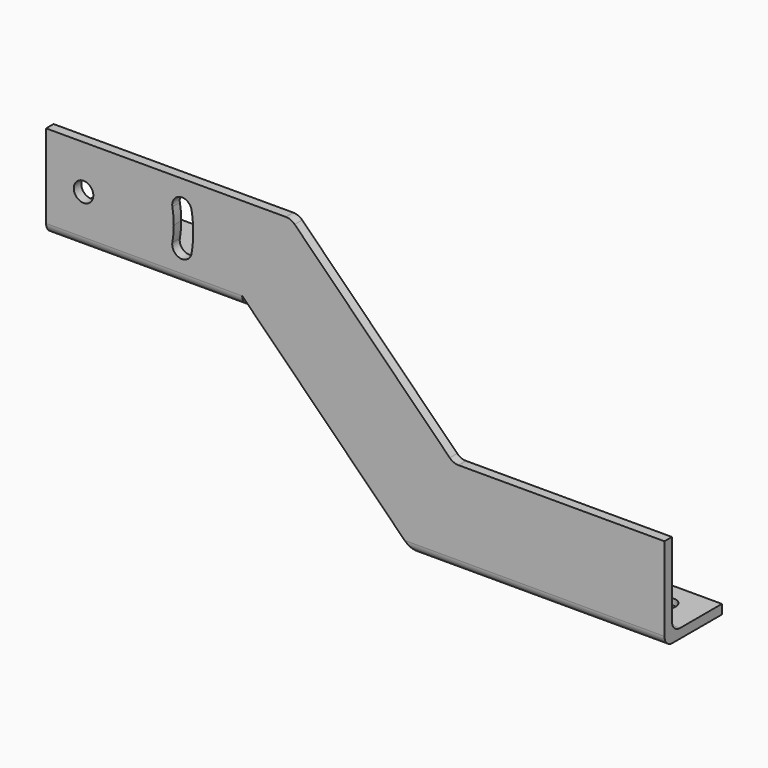
from build123d import *

# Parameters (mm, degrees)
F0_R        = 4.96062
F1_DEPTH    = 4.7625
F2_W        = 31.75
F2_H        = 4.7625
F3_DEPTH    = 127
F4_T1_DEPTH = 127
F4_T3_DEPTH = 152.4
F5_R        = 4.96062
F6_DEPTH    = 3.175
F7_W        = 31.75
F7_H        = 4.7625
F8_DEPTH    = 99.695
F9_R        = 5.08
F11_DEPTH   = 25.4


# Not quite as in the source:
# - a fillet or chamfer that OpenCascade refuses, or shapes differently, is made with other operations: its cross-section is extruded or revolved along the edge and cut away or added


with BuildPart() as f1:
    # F0 (on Front) → F1 (new body)
    with BuildSketch(Plane.XZ):
        with BuildLine():
            Line((-82.55, 82.55), (0, 0))
            Line((0, 0), (127, 0))
            Line((127, 0), (127, 47.625))
            Line((127, 47.625), (22.3571770291, 47.625))
            ThreePointArc((22.3571770291, 47.625), (19.9271372336, 48.1083649686), (17.8670489686, 49.4848719395))
            Line((17.8670489686, 49.4848719395), (-60.9632071525, 128.3151280605))
            ThreePointArc((-60.9632071525, 128.3151280605), (-63.0232954175, 129.6916350314), (-65.4533352131, 130.175))
            Line((-65.4533352131, 130.175), (-187.325, 130.175))
            Line((-187.325, 130.175), (-187.325, 82.55))
            Line((-187.325, 82.55), (-82.55, 82.55))
        make_face()
        with Locations((-168.275, 107.95)):
            Circle(F0_R, mode=Mode.SUBTRACT)
        with BuildLine():
            ThreePointArc((-113.3757178125, 117.6693530802), (-112.7358395418, 112.8283875), (-112.522, 107.95))
            ThreePointArc((-112.522, 107.95), (-112.7358395418, 103.0716125), (-113.3757178125, 98.2306469198))
            ThreePointArc((-113.3757178125, 98.2306469198), (-119.1163255014, 94.2169402337), (-123.1300321875, 99.9575479227))
            ThreePointArc((-123.1300321875, 99.9575479227), (-122.6038452724, 103.9383875), (-122.428, 107.95))
            ThreePointArc((-122.428, 107.95), (-122.6038452724, 111.9616125), (-123.1300321875, 115.9424520773))
            ThreePointArc((-123.1300321875, 115.9424520773), (-119.1163255014, 121.6830597663), (-113.3757178125, 117.6693530802))
        make_face(mode=Mode.SUBTRACT)
    extrude(amount=F1_DEPTH)

    # F2 (on face) → F3 (join)
    with BuildSketch(Plane.YZ.offset(127)):
        with Locations((15.875, 2.38125)):
            Rectangle(F2_W, F2_H)
    extrude(amount=-F3_DEPTH)

    # F4: fillet of radius 5.08 on 2 edges, made by hand

    # F4_s2 → F4_t1 (join)
    with BuildSketch(Plane.YZ):
        with BuildLine():
            ThreePointArc((5.08, 4.7625), (1.4878975516, 6.2503975516), (0, 9.8425))
            Line((0, 9.8425), (0, 4.7625))
            Line((0, 4.7625), (5.08, 4.7625))
        make_face()
    extrude(amount=F4_T1_DEPTH)

    # F4_s4 → F4_t3 (cut)
    with BuildSketch(Plane.YZ.offset(-12.7)):
        with BuildLine():
            ThreePointArc((-4.7625, 5.08), (-3.2746024484, 1.4878975516), (0.3175, 0))
            Line((0.3175, 0), (-4.7625, 0))
            Line((-4.7625, 0), (-4.7625, 5.08))
        make_face()
    extrude(amount=F4_T3_DEPTH, mode=Mode.SUBTRACT)

    # F5 (on face) → F6 (cut)
    with BuildSketch(Plane.XY.offset(4.7625)):
        with Locations((17.79778, 18.42008)):
            Circle(F5_R)
        with Locations((63.51778, 18.42008)):
            Circle(F5_R)
        with Locations((109.23778, 18.42008)):
            Circle(F5_R)
    extrude(amount=-F6_DEPTH, mode=Mode.SUBTRACT)

    # F7 (on face) → F8 (join)
    with BuildSketch(Plane(origin=(-187.325, 0, 0), x_dir=(0, -1, 0), z_dir=(-1, 0, 0))):
        with Locations((-15.875, 84.93125)):
            Rectangle(F7_W, F7_H)
    extrude(amount=-F8_DEPTH)

    # F9
    f9_edges = [f1.edges().sort_by_distance(p)[0] for p in [
        (-134.9375, -4.7625, 82.55),
        (-137.4775, 0, 87.3125),
    ]]
    fillet(f9_edges, radius=F9_R)

    # F10 (on face) → F11 (cut)
    with BuildSketch(Plane.XZ.offset(4.7625)):
        Polygon((-82.5599315833, 82.5599315833), (-87.63, 87.63), (-87.63, 82.5599315833), align=None)
    extrude(amount=-F11_DEPTH, mode=Mode.SUBTRACT)


solid = f1.part
